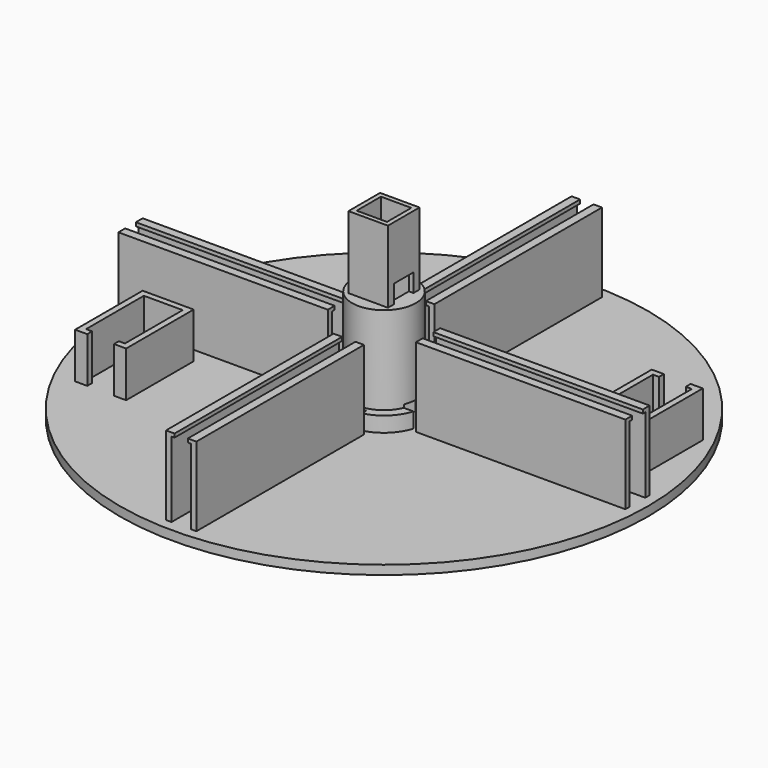
from build123d import *

# Parameters (mm, degrees)
F0_R      = 2209.8
F0_R_2    = 342.9
F0_R_3    = 266.7
F0_W      = 365.76
F0_H      = 365.76
F0_W_2    = 223.52
F0_H_2    = 50.8
F1_DEPTH  = 76.2
F0_W_3    = 355.6
F0_H_3    = 355.6
F0_W_4    = 254
F0_H_4    = 254
F2_DEPTH  = 863.6
F3_DEPTH  = 584.2
F4_W      = 330.2
F4_H      = 330.2
F4_W_2    = 254
F4_H_2    = 254
F5_DEPTH  = 604.52
F6_DEPTH  = 127
F7_W      = 203.2
F7_H      = 152.4
F8_DEPTH  = 350.52
F9_DEPTH  = 660.4
F10_W     = 111.76
F10_H     = 30.48
F11_DEPTH = 1832.356
F12_W     = 111.76
F12_H     = 31.626664176
F13_DEPTH = 1793.24
F14_W     = 111.76
F14_H     = 31.626664176
F15_DEPTH = 1833.88
F16_W     = 111.76
F16_H     = 31.626664176
F17_DEPTH = 1811.02
F18_DEPTH = 381
F19_W     = 203.2
F19_H     = 152.4
F20_DEPTH = 347.472


# Not quite as in the source:
# - a feature names something its author has since deleted; it is built from what else it names


with BuildPart() as f1:
    # F0 (on Top) → F1 (new body)
    with BuildSketch(Plane.XY):
        Circle(F0_R)
        Polygon((-1490.98, -960.12), (-1714.5, -960.12), (-1816.1, -960.12), (-1816.1, -254), (-1389.38, -254), (-1389.38, -960.12), align=None, mode=Mode.SUBTRACT)
        Polygon((127, -2120.9), (-127, -2120.9), (-127, -368.3), (-1.175e-06, -368.3), (127, -368.3), align=None, mode=Mode.SUBTRACT)
        Polygon((-368.3, 127), (-368.3, 5.095e-07), (-368.3, -127), (-2120.9, -127), (-2120.9, 127), align=None, mode=Mode.SUBTRACT)
        with BuildLine():
            ThreePointArc((368.3, 0), (260.4274270956, -260.4274279264), (-1.175e-06, -368.3))
            ThreePointArc((-1.175e-06, -368.3), (-260.4274281066, -260.4274269154), (-368.3, 5.095e-07))
            ThreePointArc((-368.3, 5.095e-07), (-260.4274272736, 260.4274277484), (1.62e-07, 368.3))
            ThreePointArc((1.62e-07, 368.3), (260.4274275683, 260.4274274537), (368.3, 0))
        make_face(mode=Mode.SUBTRACT)
        Polygon((368.3, -127), (368.3, 0), (368.3, 127), (2120.9, 127), (2120.9, -127), align=None, mode=Mode.SUBTRACT)
        Polygon((1579.88, 952.5), (1803.4, 952.5), (1905, 952.5), (1905, 254), (1478.28, 254), (1478.28, 952.5), align=None, mode=Mode.SUBTRACT)
        Polygon((127, 368.3), (1.62e-07, 368.3), (-127, 368.3), (-127, 2120.9), (127, 2120.9), align=None, mode=Mode.SUBTRACT)
        Polygon((-127, 368.3), (1.62e-07, 368.3), (127, 368.3), (127, 2120.9), (-127, 2120.9), align=None)
        Polygon((368.3, 127), (368.3, 0), (368.3, -127), (2120.9, -127), (2120.9, 127), align=None)
        Polygon((-368.3, -127), (-368.3, 5.095e-07), (-368.3, 127), (-2120.9, 127), (-2120.9, -127), align=None)
        Polygon((-127, -368.3), (-127, -2120.9), (127, -2120.9), (127, -368.3), (-1.175e-06, -368.3), align=None)
        with BuildLine():
            ThreePointArc((-368.3, 5.095e-07), (-260.4274281066, -260.4274269154), (-1.175e-06, -368.3))
            ThreePointArc((-1.175e-06, -368.3), (260.4274270956, -260.4274279264), (368.3, 0))
            ThreePointArc((368.3, 0), (260.4274275683, 260.4274274537), (1.62e-07, 368.3))
            ThreePointArc((1.62e-07, 368.3), (-260.4274272736, 260.4274277484), (-368.3, 5.095e-07))
        make_face()
        Circle(F0_R_2, mode=Mode.SUBTRACT)
        Circle(F0_R_2)
        Circle(F0_R_3, mode=Mode.SUBTRACT)
        Circle(F0_R_3)
        Rectangle(F0_W, F0_H, mode=Mode.SUBTRACT)
        Polygon((-1440.18, -304.8), (-1765.3, -304.8), (-1765.3, -909.32), (-1714.5, -909.32), (-1490.98, -909.32), (-1440.18, -909.32), align=None)
        Polygon((1529.08, 304.8), (1854.2, 304.8), (1854.2, 901.7), (1803.4, 901.7), (1579.88, 901.7), (1529.08, 901.7), align=None)
        Polygon((-1765.3, -909.32), (-1765.3, -304.8), (-1440.18, -304.8), (-1440.18, -909.32), (-1490.98, -909.32), (-1490.98, -960.12), (-1389.38, -960.12), (-1389.38, -254), (-1816.1, -254), (-1816.1, -960.12), (-1714.5, -960.12), (-1714.5, -909.32), align=None)
        Polygon((1854.2, 901.7), (1854.2, 304.8), (1529.08, 304.8), (1529.08, 901.7), (1579.88, 901.7), (1579.88, 952.5), (1478.28, 952.5), (1478.28, 254), (1905, 254), (1905, 952.5), (1803.4, 952.5), (1803.4, 901.7), align=None)
        with Locations((1691.64, 927.1)):
            Rectangle(F0_W_2, F0_H_2)
        with Locations((-1602.74, -934.72)):
            Rectangle(F0_W_2, F0_H_2)
    extrude(amount=-F1_DEPTH)

    # F0 (on Top) → F2 (join)
    with BuildSketch(Plane.XY):
        Circle(F0_R_3)
        Rectangle(F0_W, F0_H, mode=Mode.SUBTRACT)
        Rectangle(F0_W, F0_H)
        Rectangle(F0_W_3, F0_H_3, mode=Mode.SUBTRACT)
        Rectangle(F0_W_3, F0_H_3)
        Rectangle(F0_W_4, F0_H_4, mode=Mode.SUBTRACT)
    extrude(amount=F2_DEPTH)

    # F0 (on Top) → F3 (cut)
    with BuildSketch(Plane.XY):
        Rectangle(F0_W, F0_H)
        Rectangle(F0_W_3, F0_H_3, mode=Mode.SUBTRACT)
        Rectangle(F0_W_3, F0_H_3)
        Rectangle(F0_W_4, F0_H_4, mode=Mode.SUBTRACT)
        Rectangle(F0_W_4, F0_H_4)
    extrude(amount=F3_DEPTH, mode=Mode.SUBTRACT)

    # F4 (on face) → F5 (join)
    with BuildSketch(Plane.XY.offset(863.6)):
        Rectangle(F4_W, F4_H)
        Rectangle(F4_W_2, F4_H_2, mode=Mode.SUBTRACT)
    extrude(amount=F5_DEPTH)

    # F0 (on Top) → F6 (join)
    with BuildSketch(Plane.XY):
        Circle(F0_R_2)
        Circle(F0_R_3, mode=Mode.SUBTRACT)
    extrude(amount=F6_DEPTH)

    # F7 (on Right) → F8 (cut, symmetric)
    with BuildSketch(Plane.YZ):
        with Locations((0, 76.2)):
            Rectangle(F7_W, F7_H)
    extrude(amount=F8_DEPTH, both=True, mode=Mode.SUBTRACT)

    # F0 (on Top) → F9 (join)
    with BuildSketch(Plane.XY):
        Polygon((-127, -368.3), (-127, -2120.9), (127, -2120.9), (127, -368.3), (-1.175e-06, -368.3), align=None)
        Polygon((-368.3, -127), (-368.3, 5.095e-07), (-368.3, 127), (-2120.9, 127), (-2120.9, -127), align=None)
        Polygon((-127, 368.3), (1.62e-07, 368.3), (127, 368.3), (127, 2120.9), (-127, 2120.9), align=None)
        Polygon((368.3, 127), (368.3, 0), (368.3, -127), (2120.9, -127), (2120.9, 127), align=None)
    extrude(amount=F9_DEPTH)

    # F10 (on face) → F11 (cut)
    with BuildSketch(Plane.XZ.offset(2120.9)):
        Polygon((-55.88, 629.92), (-81.28, 629.92), (-81.28, 0), (81.28, 0), (81.28, 629.92), (55.88, 629.92), align=None)
        with Locations((0, 645.16)):
            Rectangle(F10_W, F10_H)
    extrude(amount=-F11_DEPTH, mode=Mode.SUBTRACT)

    # F12 (on face) → F13 (cut)
    with BuildSketch(Plane(origin=(-2120.9, 0, 0), x_dir=(0, -1, 0), z_dir=(-1, 0, 0))):
        Polygon((-55.88, 629.92), (-81.28, 629.92), (-81.28, 0), (81.28, 0), (81.28, 629.92), (55.88, 629.92), align=None)
        with Locations((0, 645.733332088)):
            Rectangle(F12_W, F12_H)
    extrude(amount=-F13_DEPTH, mode=Mode.SUBTRACT)

    # F14 (on face) → F15 (cut)
    with BuildSketch(Plane(origin=(0, 2120.9, 0), x_dir=(-1, 0, 0), z_dir=(0, 1, 0))):
        Polygon((-55.88, 629.92), (-81.28, 629.92), (-81.28, 0), (81.28, 0), (81.28, 629.92), (55.88, 629.92), align=None)
        with Locations((0, 645.733332088)):
            Rectangle(F14_W, F14_H)
    extrude(amount=-F15_DEPTH, mode=Mode.SUBTRACT)

    # F16 (on face) → F17 (cut)
    with BuildSketch(Plane.YZ.offset(2120.9)):
        Polygon((-55.88, 629.92), (-81.28, 629.92), (-81.28, 0), (81.28, 0), (81.28, 629.92), (55.88, 629.92), align=None)
        with Locations((0, 645.733332088)):
            Rectangle(F16_W, F16_H)
    extrude(amount=-F17_DEPTH, mode=Mode.SUBTRACT)

    # F0 (on Top) → F18 (join)
    with BuildSketch(Plane.XY):
        Polygon((-1765.3, -909.32), (-1765.3, -304.8), (-1440.18, -304.8), (-1440.18, -909.32), (-1490.98, -909.32), (-1490.98, -960.12), (-1389.38, -960.12), (-1389.38, -254), (-1816.1, -254), (-1816.1, -960.12), (-1714.5, -960.12), (-1714.5, -909.32), align=None)
        Polygon((1854.2, 901.7), (1854.2, 304.8), (1529.08, 304.8), (1529.08, 901.7), (1579.88, 901.7), (1579.88, 952.5), (1478.28, 952.5), (1478.28, 254), (1905, 254), (1905, 952.5), (1803.4, 952.5), (1803.4, 901.7), align=None)
    extrude(amount=F18_DEPTH)

    # F19 (on face) → F20 (cut)
    with BuildSketch(Plane.YZ.offset(165.1)):
        with Locations((0, 939.8)):
            Rectangle(F19_W, F19_H)
    extrude(amount=-F20_DEPTH, mode=Mode.SUBTRACT)


solid = f1.part
